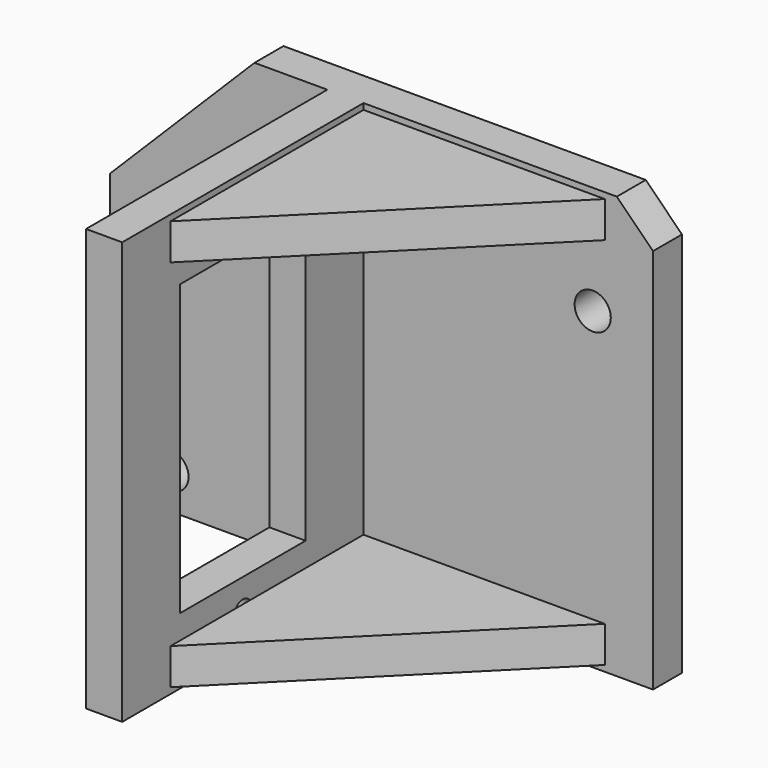
from build123d import *

# Parameters (mm, degrees)
F0_R        = 1.5
F1_DEPTH    = 3
F2_W        = 3
F2_H        = 35
F3_DEPTH    = 25
F4_W        = 13
F4_H        = 24
F4_R        = 0.875
F5_DEPTH    = 27.001
F6_W        = 20
F6_H        = 3
F7_DEPTH    = 23
F8_T4_DEPTH = 121.2974174464


# Not quite as in the source:
# - a fillet or chamfer that OpenCascade refuses, or shapes differently, is made with other operations: its cross-section is extruded or revolved along the edge and cut away or added
# - a feature of the source that left no trace in its solid (it failed there, or was rolled back) is left out


with BuildPart() as f1:
    # F0 (on Front) → F1 (new body)
    with BuildSketch(Plane.XZ):
        Polygon((-19.1084720148, 23.034380586), (-19.1084720148, 0), (25.8915279852, 0), (25.8915279852, 32), (22.8915279852, 35), (-7.1428526009, 35), align=None)
        with Locations((-14.1084720148, 3)):
            Circle(F0_R, mode=Mode.SUBTRACT)
        with Locations((20.8915279852, 26)):
            Circle(F0_R, mode=Mode.SUBTRACT)
    extrude(amount=F1_DEPTH)

    # F2 (on face) → F3 (join)
    with BuildSketch(Plane.XZ.offset(3)):
        with Locations((0.3915279852, 17.5)):
            Rectangle(F2_W, F2_H)
    extrude(amount=F3_DEPTH)

    # F4 (on face) → F5 (cut, through all)
    with BuildSketch(Plane(origin=(-1.1084720148, 0, 0), x_dir=(0, -1, 0), z_dir=(-1, 0, 0))):
        with Locations((15.5, 17.5)):
            Rectangle(F4_W, F4_H)
        with Locations((15.5, 32)):
            Circle(F4_R)
        with Locations((15.5, 3)):
            Circle(F4_R)
    extrude(amount=-F5_DEPTH, mode=Mode.SUBTRACT)

    # F6 (on face) → F7 (join)
    with BuildSketch(Plane.XZ.offset(3)):
        with Locations((11.8915279852, 33)):
            Rectangle(F6_W, F6_H)
        with Locations((11.8915279852, 2)):
            Rectangle(F6_W, F6_H)
    extrude(amount=F7_DEPTH)

    # F8: chamfer of 23 on 1 edges, made by hand


with BuildPart() as f8_tool2:
    # F8_s3 → F8_t4 (new body)
    with BuildSketch(Plane.XY.offset(-58.6487087232)):
        Polygon((21.8915279852, -3), (-1.1084720148, -26), (21.8915279852, -26), align=None)
    extrude(amount=F8_T4_DEPTH)

    split(bisect_by=Plane.XZ.offset(3), keep=Keep.TOP)

    split(bisect_by=Plane.YZ.offset(1.8915279852), keep=Keep.TOP)


with BuildPart() as f1_1:
    add(f1.part)

    # F8_t1: cut F8_tool2
    add(f8_tool2.part, mode=Mode.SUBTRACT)


solid = f1_1.part
